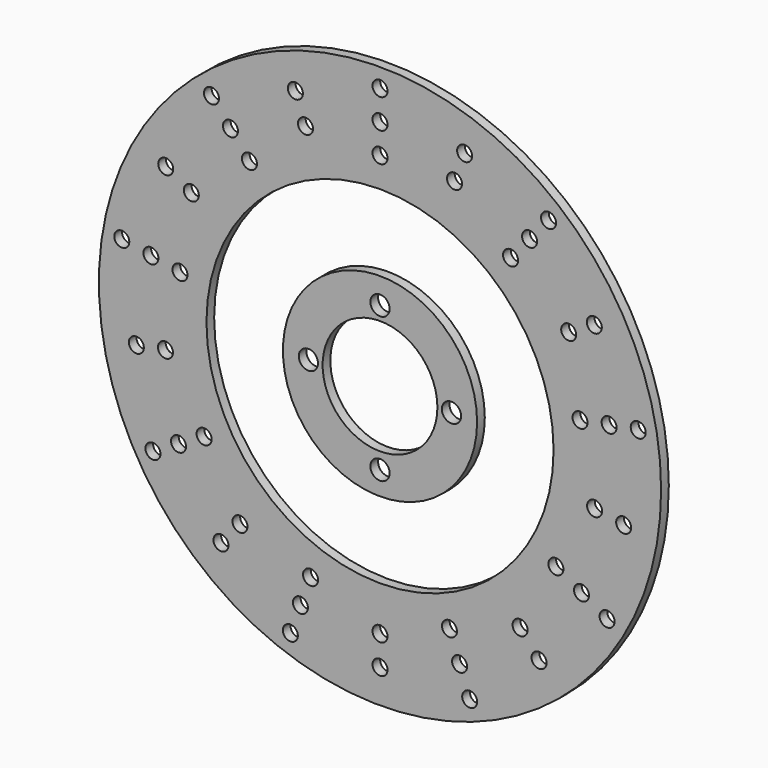
from build123d import *

# Parameters (mm, degrees)
F0_R            = 148.3741
F0_R_2          = 91.6051
F3_DEPTH        = 5.08
F2_R            = 3.9624
F4_DEPTH        = 5.081
F4_COPIES_COUNT = 9
F6_D            = 7.9248
F6_COPIES_COUNT = 9
F0_R_3          = 51.2445
F0_R_4          = 30.2895
F7_DEPTH        = 5.08
F8_D            = 10.16


# Not quite as in the source:
# - a pattern or mirror of a feature is missing from the dataset's text; its kind, count and spacing are read off the source's solid


with BuildPart() as f3:
    # F0 (on Front) → F3 (new body)
    with BuildSketch(Plane.XZ):
        Circle(F0_R)
        Circle(F0_R_2, mode=Mode.SUBTRACT)
    extrude(amount=F3_DEPTH)

    # F2 (on face) → F4 (cut, through all)
    with BuildSketch(Plane.XZ):
        with Locations((0, 107.2007)):
            Circle(F2_R)
        with Locations((0, 122.7963)):
            Circle(F2_R)
        with Locations((0, 138.3919)):
            Circle(F2_R)
    f4 = extrude(amount=F4_DEPTH, mode=Mode.SUBTRACT)

    # F4_copies: F4 ×9 about axis
    f4_copies_axis = Axis((0, 0, 0), (0, 1, 0))
    for i in range(1, F4_COPIES_COUNT):
        add(f4.rotate(f4_copies_axis, i * 360 / F4_COPIES_COUNT), mode=Mode.SUBTRACT)

    # F6 (through all)
    with Locations(Plane(origin=(0, 0, 0), x_dir=(1, 0, 0), z_dir=(0, 1, 0))):
        with Locations((0, 114.9985), (0, 130.5941)):
            f6 = Hole(F6_D / 2)

    # F6_copies: F6 ×9 about axis
    f6_copies_axis = Axis((0, 0, 0), (0, 1, 0))
    for i in range(1, F6_COPIES_COUNT):
        add(f6.rotate(f6_copies_axis, i * 360 / F6_COPIES_COUNT), mode=Mode.SUBTRACT)


with BuildPart() as f7:
    # F0 (on Front) → F7 (new body)
    with BuildSketch(Plane.XZ):
        Circle(F0_R_3)
        Circle(F0_R_4, mode=Mode.SUBTRACT)
    extrude(amount=F7_DEPTH)

    # F8 (through all)
    with Locations(Plane(origin=(0, 0, 0), x_dir=(1, 0, 0), z_dir=(0, 1, 0))):
        with Locations((0, -37.5412), (37.7119863628, 0), (0, 38.8407654956), (-37.8069085799, 0)):
            Hole(F8_D / 2)


solid = Compound([f3.part, f7.part])
